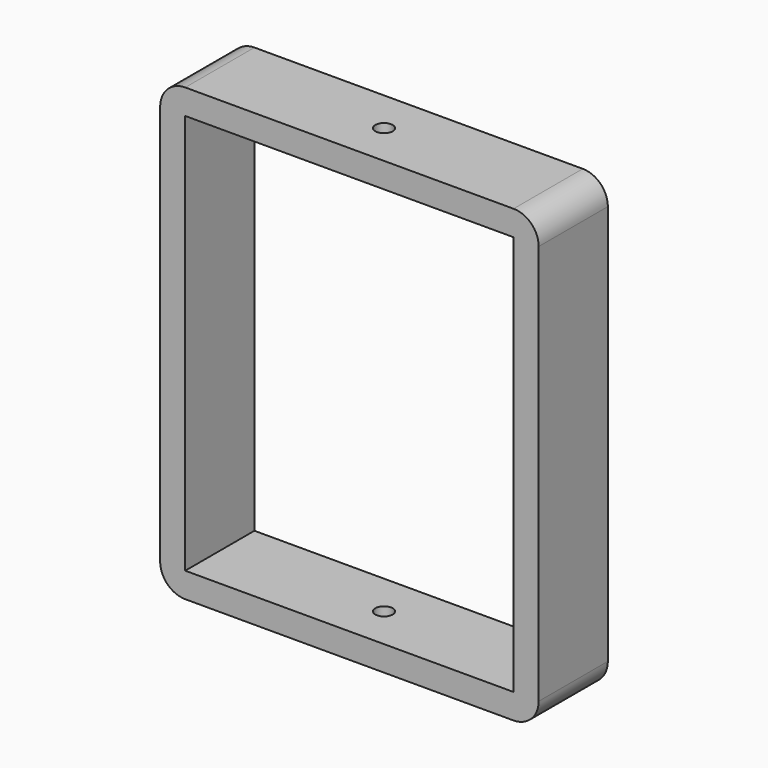
from build123d import *

# Parameters (mm, degrees)
F1_DEPTH = 25
F3_R     = 2.5
F4_DEPTH = 25
F2_R     = 2.5
F5_DEPTH = 25


# Not quite as in the source:
# - ends of sketch curves that miss each other by under 0.0002 mm in the source are joined


with BuildPart() as f1:
    # F0 (on Front) → F1 (new body)
    with BuildSketch(Plane.XZ):
        with BuildLine():
            Line((-47.4549531937, 57.8603595495), (47.4549531937, 57.8603595495))
            Line((47.4549531937, 57.8603595495), (47.4549531937, 65.1126131415))
            Line((47.4549531937, 65.1126131415), (-47.4549531937, 65.1126131415))
            ThreePointArc((-47.4549531937, 65.1126131415), (-52.5830735216, 62.9884798775), (-54.707210511, 57.8603595495))
            Line((-54.707210511, 57.8603595495), (-54.7072067857, -57.8603595495))
            ThreePointArc((-54.7072067857, -57.8603595495), (-52.5830708875, -62.9884772433), (-47.4549531937, -65.1126131415))
            Line((-47.4549531937, -65.1126131415), (-47.4549531937, -57.8603595495))
            Line((-47.4549531937, -57.8603595495), (-47.4549531937, 57.8603595495))
        make_face()
        with BuildLine():
            Line((47.4549531937, 65.1126131415), (47.4549531937, 57.8603595495))
            Line((47.4549531937, 57.8603595495), (47.4549531937, -57.8603595495))
            Line((47.4549531937, -57.8603595495), (-47.4549531937, -57.8603595495))
            Line((-47.4549531937, -57.8603595495), (-47.4549531937, -65.1126131415))
            Line((-47.4549531937, -65.1126131415), (47.4549531937, -65.1126131415))
            ThreePointArc((47.4549531937, -65.1126131415), (52.5830735216, -62.9884798775), (54.707210511, -57.8603595495))
            Line((54.707210511, -57.8603595495), (54.7072067857, 57.8603595495))
            ThreePointArc((54.7072067857, 57.8603595495), (52.5830708875, 62.9884772433), (47.4549531937, 65.1126131415))
        make_face()
    extrude(amount=F1_DEPTH)

    # F3 (on face) → F4 (cut)
    with BuildSketch(Plane(origin=(0, 0, -65.1126131415), x_dir=(1, 0, 0), z_dir=(0, 0, -1))):
        with Locations((0, 12.5)):
            Circle(F3_R)
    extrude(amount=-F4_DEPTH, mode=Mode.SUBTRACT)

    # F2 (on face) → F5 (cut)
    with BuildSketch(Plane.XY.offset(65.1126131415)):
        with Locations((0, -12.5)):
            Circle(F2_R)
    extrude(amount=-F5_DEPTH, mode=Mode.SUBTRACT)


solid = f1.part
